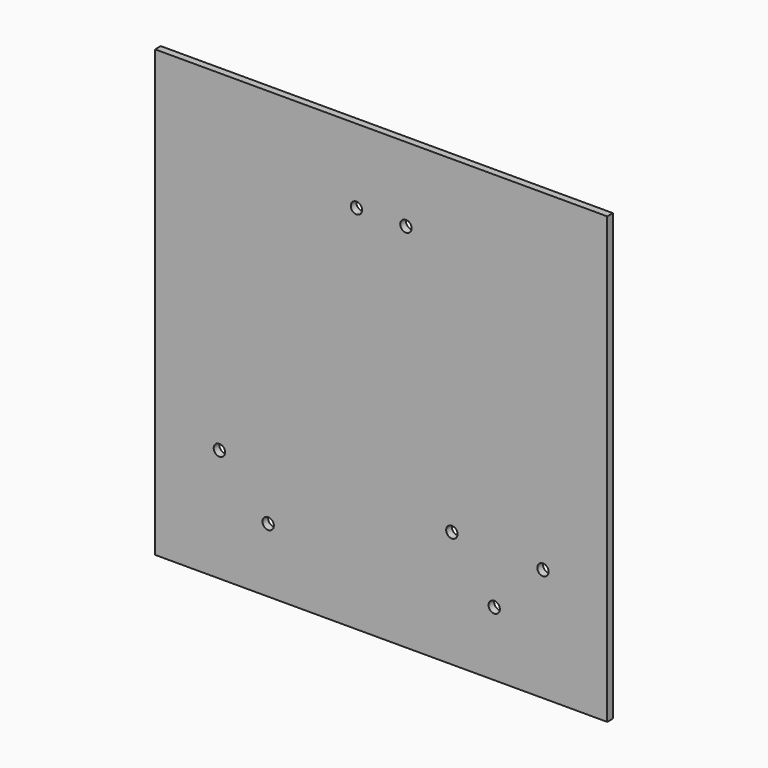
from build123d import *

# Parameters (mm, degrees)
F0_W     = 203.2
F0_H     = 200.025
F1_DEPTH = 3.175
F3_D     = 5.1054
F3_DEPTH = 25
F3_TIP   = 1.5338169022


# Not quite as in the source:
# - a length typed as a fraction of an inch, garbled in the dataset ("3 / 203.2 mm" for 3/8 in), is restored


with BuildPart() as f1:
    # F0 (on Front) → F1 (new body)
    with BuildSketch(Plane.XZ):
        Rectangle(F0_W, F0_H)
    extrude(amount=F1_DEPTH)

    # F3
    with Locations(Plane.XZ.offset(3.175)):
        with Locations((-72.7075, -49.2125), (72.7075, -49.2125), (-50.8, -71.12), (50.8, -71.12), (31.75, -47.625), (-11.1125, 66.675), (11.1125, 66.675)):
            Hole(F3_D / 2, depth=F3_DEPTH)
            with Locations((0, 0, -(F3_DEPTH + F3_TIP / 2))):  # 118° drill point
                Cone(0, F3_D / 2, F3_TIP, mode=Mode.SUBTRACT)


solid = f1.part
